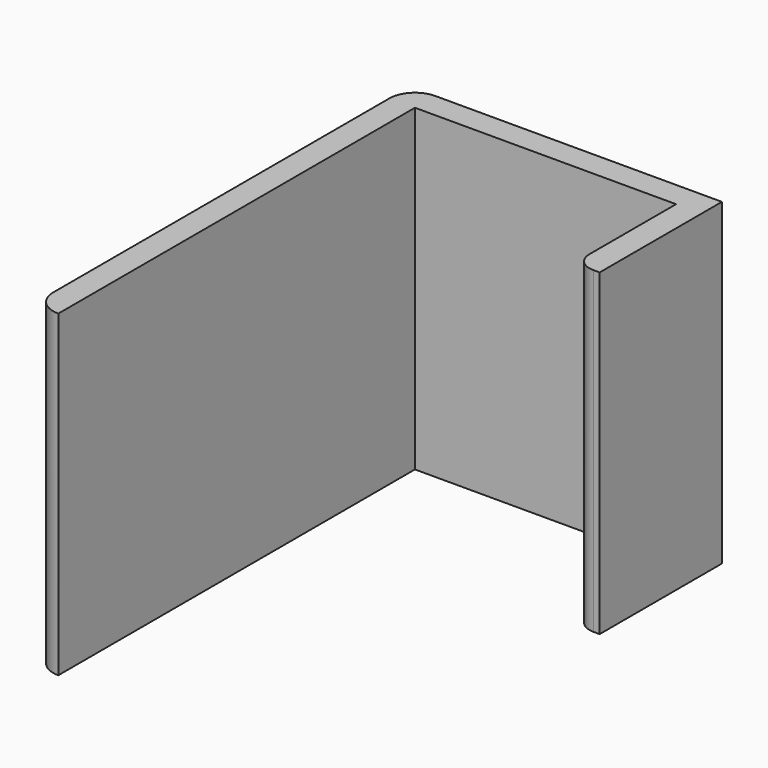
from build123d import *

# Parameters (mm, degrees)
F1_DEPTH = 25
F2_R     = 1.5
F3_R     = 1.99999


# Not quite as in the source:
# - a fillet or chamfer is up to 0.001 mm smaller than in the source, because OpenCascade refuses the exact size


with BuildPart() as f1:
    # F0 (on Top) → F1 (new body)
    with BuildSketch(Plane.XY):
        Polygon((24.5, 0), (0, 0), (0, -37), (2, -37), (2, -2), (22.5, -2), (22.5, -12), (24.5, -12), align=None)
    extrude(amount=F1_DEPTH)

    # F2
    f2_edges = [f1.edges().sort_by_distance(p)[0] for p in [
        (22.5, -12, 12.5),
    ]]
    fillet(f2_edges, radius=F2_R)

    # F3 (radius 2 in the source; OpenCascade refuses exactly that, so slightly less here)
    f3_edges = [f1.edges().sort_by_distance(p)[0] for p in [
        (0, 0, 12.5),
        (0, -37, 12.5),
    ]]
    fillet(f3_edges, radius=F3_R)


solid = f1.part
